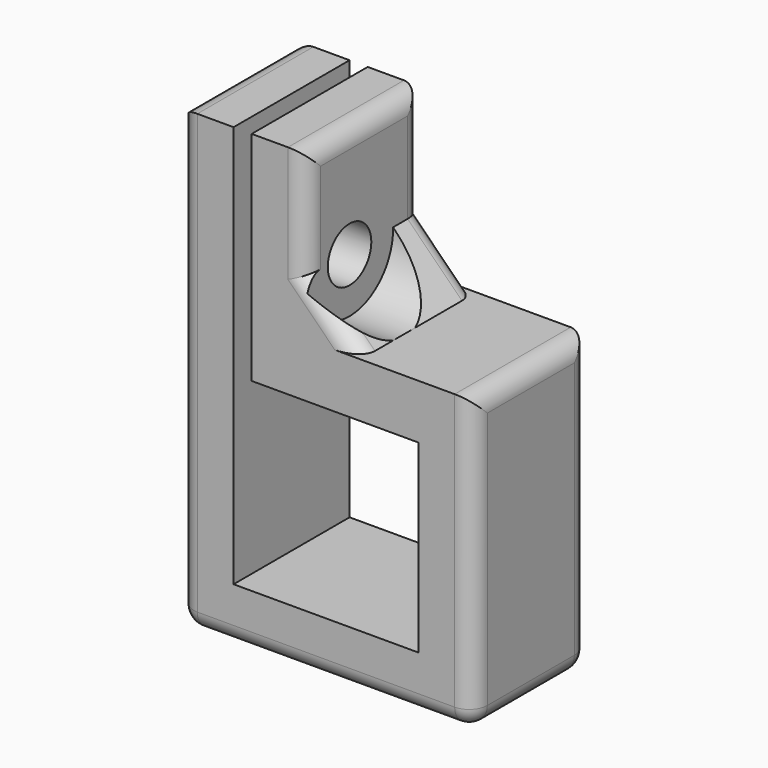
from build123d import *

# Parameters (mm, degrees)
F1_DEPTH    = 8
F2_R        = 1.5
F3_DEPTH    = 7.001
F4_T4_DEPTH = 8
F4_S5_R     = 1.5
F4_T6_DEPTH = 6
F5_R        = 1
F6_R        = 1
F7_R        = 3
F8_DEPTH    = 3


# Not quite as in the source:
# - a fillet or chamfer that OpenCascade refuses, or shapes differently, is made with other operations: its cross-section is extruded or revolved along the edge and cut away or added


with BuildPart() as f1:
    # F0 (on Front) → F1 (new body)
    with BuildSketch(Plane.XZ):
        Polygon((5.1, 5.1), (5.1, -5.1), (-5.1, -5.1), (-5.1, 5.1), (-5.1, 8.1), (-5.1, 17.1), (-8.1, 17.1), (-8.1, 8.1), (-8.1, -8.1), (8.1, -8.1), (8.1, 8.1), (-1.1, 8.1), (-1.1, 17.1), (-4.1, 17.1), (-4.1, 8.1), (-4.1, 5.1), align=None)
    extrude(amount=F1_DEPTH)

    # F2 (on face) → F3 (cut, through all)
    with BuildSketch(Plane.YZ.offset(-1.1)):
        with Locations((-5, 11)):
            Circle(F2_R)
    extrude(amount=-F3_DEPTH, mode=Mode.SUBTRACT)

    # F4: chamfer of 3 on 1 edges, made by hand


with BuildPart() as f4_tool2:
    # F4_s3 → F4_t4 (new body)
    with BuildSketch(Plane.XZ):
        Polygon((1.9, 8.1), (-1.1, 11.1), (-1.1, 8.1), align=None)
    extrude(amount=F4_T4_DEPTH)

    # F4_s5 → F4_t6 (cut, symmetric)
    with BuildSketch(Plane.YZ.offset(0.4)):
        with Locations((-5, 11)):
            Circle(F4_S5_R)
    extrude(amount=F4_T6_DEPTH, both=True, mode=Mode.SUBTRACT)


with BuildPart() as f1_1:
    add(f1.part)

    # F4_t1: union F4_tool2
    add(f4_tool2.part)

    # F5
    f5_edges = [f1_1.edges().sort_by_distance(p)[0] for p in [
        (8.1, -4, -8.1),
        (8.1, -4, 8.1),
        (8.1, 0, 0),
        (8.1, -8, 0),
        (-8.1, -4, -8.1),
        (0, 0, -8.1),
        (0, -8, -8.1),
        (-8.1, -4, 17.1),
        (-8.1, 0, 4.5),
        (-8.1, -8, 4.5),
        (-1.1, -4, 17.1),
        (-1.1, 0, 14.1),
        (-1.1, -8, 14.1),
    ]]
    fillet(f5_edges, radius=F5_R)

    # F6
    f6_edges = [f1_1.edges().sort_by_distance(p)[0] for p in [
        (0.4, 0, 9.6),
        (0.4, -8, 9.6),
    ]]
    fillet(f6_edges, radius=F6_R)

    # F7 (on face) → F8 (cut)
    with BuildSketch(Plane.YZ.offset(-1.1)):
        with Locations((-5, 11)):
            Circle(F7_R)
    extrude(amount=F8_DEPTH, mode=Mode.SUBTRACT)


solid = f1_1.part
